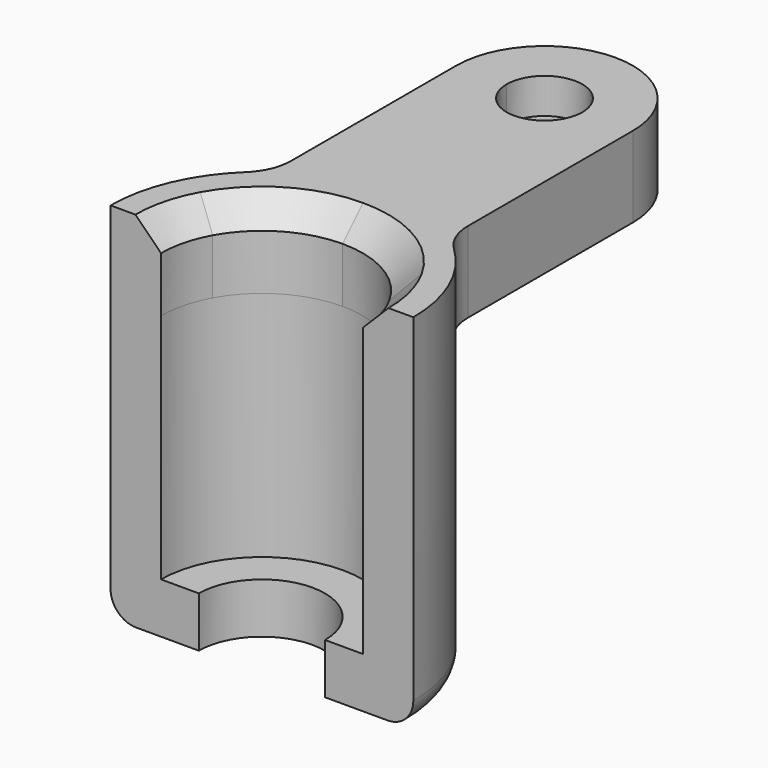
from build123d import *

# Parameters (mm, degrees)
F1_DEPTH    = 2
F2_DEPTH    = 25
F4_DEPTH    = 8
F5_DEPTH    = 4.5
F6_T1_DEPTH = 8
F7_DEPTH    = 3
F8_R        = 2.54
F9_SIZE     = 2.54


# Not quite as in the source:
# - a fillet or chamfer that OpenCascade refuses, or shapes differently, is made with other operations: its cross-section is extruded or revolved along the edge and cut away or added


with BuildPart() as f1:
    # F0 (on Top) → F1 (new body)
    with BuildSketch(Plane.XY):
        with BuildLine():
            Line((6.25, 0), (10, 0))
            ThreePointArc((10, 0), (0, 10), (-10, 0))
            Line((-10, 0), (-6.25, 0))
            ThreePointArc((-6.25, 0), (0, 6.25), (6.25, 0))
        make_face()
    extrude(amount=F1_DEPTH)

    # F0 (on Top) → F2 (join)
    with BuildSketch(Plane.XY):
        with BuildLine():
            ThreePointArc((-10, 0), (0, 10), (10, 0))
            Line((10, 0), (15, 0))
            ThreePointArc((15, 0), (0, 15), (-15, 0))
            Line((-15, 0), (-10, 0))
        make_face()
    extrude(amount=F2_DEPTH)

    # F3 (on face) → F4 (join)
    with BuildSketch(Plane.XY.offset(25)):
        with BuildLine():
            ThreePointArc((-8.75, 12.183492931), (-4.5960638613, 14.2785222268), (0, 15))
            Line((0, 15), (0, 26.25))
            ThreePointArc((0, 26.25), (-6.1871843354, 28.8128156646), (-8.75, 35))
            Line((-8.75, 35), (-8.75, 12.183492931))
        make_face()
        with BuildLine():
            Line((0, 26.25), (0, 15))
            ThreePointArc((0, 15), (4.5960638613, 14.2785222268), (8.75, 12.183492931))
            Line((8.75, 12.183492931), (8.75, 35))
            ThreePointArc((8.75, 35), (6.1871843354, 28.8128156646), (0, 26.25))
        make_face()
        with BuildLine():
            ThreePointArc((8.75, 35), (0, 43.75), (-8.75, 35))
            Line((-8.75, 35), (-3.75, 35))
            ThreePointArc((-3.75, 35), (0, 38.75), (3.75, 35))
            Line((3.75, 35), (8.75, 35))
        make_face()
        with BuildLine():
            Line((8.75, 12.183492931), (8.75, 4.8412291828))
            ThreePointArc((8.75, 4.8412291828), (9.6824583655, 2.5), (10, 0))
            Line((10, 0), (15, 0))
            ThreePointArc((15, 0), (13.346347815, 6.8465319688), (8.75, 12.183492931))
        make_face()
        with BuildLine():
            ThreePointArc((-10, 0), (-9.6824583655, 2.5), (-8.75, 4.8412291828))
            Line((-8.75, 4.8412291828), (-8.75, 12.183492931))
            ThreePointArc((-8.75, 12.183492931), (-13.346347815, 6.8465319688), (-15, 0))
            Line((-15, 0), (-10, 0))
        make_face()
        with BuildLine():
            Line((0, 15), (0, 10))
            ThreePointArc((0, 10), (5.0787650158, 8.6142989218), (8.75, 4.8412291828))
            Line((8.75, 4.8412291828), (8.75, 12.183492931))
            ThreePointArc((8.75, 12.183492931), (4.5960638613, 14.2785222268), (0, 15))
        make_face()
        with BuildLine():
            ThreePointArc((-8.75, 4.8412291828), (-5.0787650158, 8.6142989218), (0, 10))
            Line((0, 10), (0, 15))
            ThreePointArc((0, 15), (-4.5960638613, 14.2785222268), (-8.75, 12.183492931))
            Line((-8.75, 12.183492931), (-8.75, 4.8412291828))
        make_face()
        with BuildLine():
            ThreePointArc((-8.75, 35), (-6.1871843354, 28.8128156646), (0, 26.25))
            Line((0, 26.25), (0, 31.25))
            ThreePointArc((0, 31.25), (-2.6516504294, 32.3483495706), (-3.75, 35))
            Line((-3.75, 35), (-8.75, 35))
        make_face()
        with BuildLine():
            Line((0, 31.25), (0, 26.25))
            ThreePointArc((0, 26.25), (6.1871843354, 28.8128156646), (8.75, 35))
            Line((8.75, 35), (3.75, 35))
            ThreePointArc((3.75, 35), (2.6516504294, 32.3483495706), (0, 31.25))
        make_face()
    extrude(amount=F4_DEPTH)

    # F3 (on face) → F5 (join)
    with BuildSketch(Plane.XY.offset(25)):
        with BuildLine():
            ThreePointArc((3.75, 35), (0, 38.75), (-3.75, 35))
            Line((-3.75, 35), (-2.25, 35))
            ThreePointArc((-2.25, 35), (0, 37.25), (2.25, 35))
            Line((2.25, 35), (3.75, 35))
        make_face()
        with BuildLine():
            ThreePointArc((-3.75, 35), (-2.6516504294, 32.3483495706), (0, 31.25))
            Line((0, 31.25), (0, 32.75))
            ThreePointArc((0, 32.75), (-1.5909902577, 33.4090097423), (-2.25, 35))
            Line((-2.25, 35), (-3.75, 35))
        make_face()
        with BuildLine():
            Line((0, 32.75), (0, 31.25))
            ThreePointArc((0, 31.25), (2.6516504294, 32.3483495706), (3.75, 35))
            Line((3.75, 35), (2.25, 35))
            ThreePointArc((2.25, 35), (1.5909902577, 33.4090097423), (0, 32.75))
        make_face()
    extrude(amount=F5_DEPTH)

    # F6: fillet of radius 5.08 on 2 edges, made by hand

    # F6_s2 → F6_t1 (join)
    with BuildSketch(Plane.XY.offset(25)):
        with BuildLine():
            ThreePointArc((-10.3311752988, 10.8750548019), (-9.1620009917, 12.5540311317), (-8.75, 14.5580733615))
            Line((-8.75, 14.5580733615), (-8.75, 12.183492931))
            ThreePointArc((-8.75, 12.183492931), (-9.5629919628, 11.5563482433), (-10.3311752988, 10.8750548019))
        make_face()
        with BuildLine():
            ThreePointArc((10.3311752988, 10.8750548019), (9.1620009917, 12.5540311317), (8.75, 14.5580733615))
            Line((8.75, 14.5580733615), (8.75, 12.183492931))
            ThreePointArc((8.75, 12.183492931), (9.5629919628, 11.5563482433), (10.3311752988, 10.8750548019))
        make_face()
    extrude(amount=F6_T1_DEPTH)

    # F7 (add): a face of the model
    f7_faces = [f1.faces().sort_by_distance(p)[0] for p in [
        (0, 7.1463690133, 0),
    ]]
    extrude(f7_faces, amount=F7_DEPTH)

    # F8
    f8_edges = [f1.edges().sort_by_distance(p)[0] for p in [
        (0, 15, -3),
    ]]
    fillet(f8_edges, radius=F8_R)

    # F9
    f9_edges = [f1.edges().sort_by_distance(p)[0] for p in [
        (0, 10, 33),
    ]]
    chamfer(f9_edges, length=F9_SIZE)


solid = f1.part
